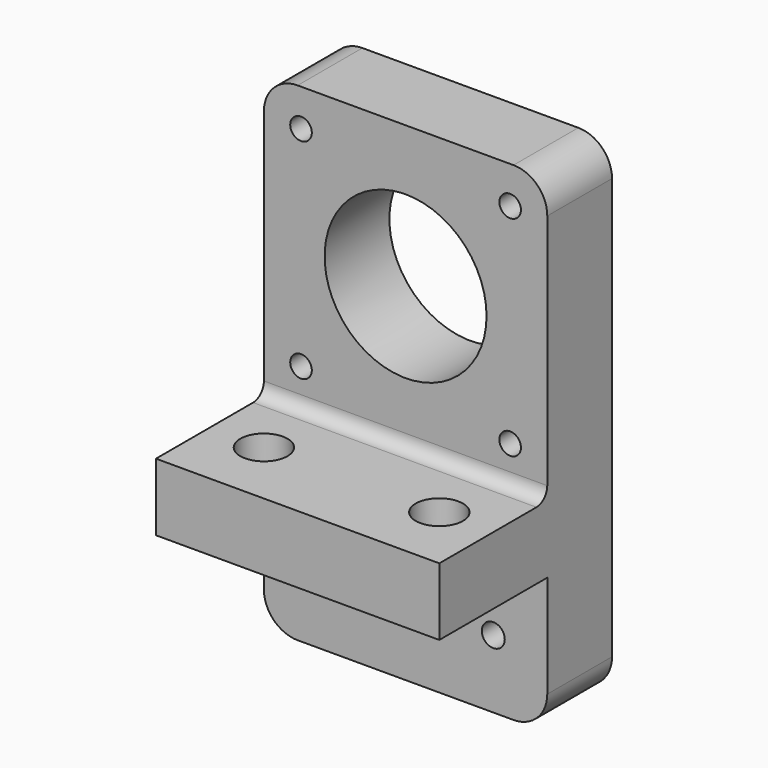
from build123d import *

# Parameters (mm, degrees)
F0_W     = 42
F0_H     = 10
F1_DEPTH = 20
F0_H_2   = 42
F0_R     = 1.6
F0_R_2   = 12
F0_H_3   = 20.2
F0_R_3   = 3.5
F0_H_4   = 0.1999993771
F2_DEPTH = 12
F3_R     = 1.7
F4_DEPTH = 25
F3_R_2   = 3.5
F5_DEPTH = 4
F0_R_4   = 1.7
F6_DEPTH = 12
F7_R     = 3.5
F7_R_2   = 1.7
F8_DEPTH = 2
F9_R     = 5
F10_R    = 2


# Not quite as in the source:
# - a feature names something its author has since deleted; it is built from what else it names


with BuildPart() as f1:
    # F0 (on Front) → F1 (new body)
    with BuildSketch(Plane.XZ):
        with Locations((0, -26.1999993771)):
            Rectangle(F0_W, F0_H)
    extrude(amount=F1_DEPTH)

    # F0 (on Front) → F2 (join)
    with BuildSketch(Plane.XZ):
        Rectangle(F0_W, F0_H_2)
        with Locations((-15.5, -15.5)):
            Circle(F0_R, mode=Mode.SUBTRACT)
        with Locations((15.5, -15.5)):
            Circle(F0_R, mode=Mode.SUBTRACT)
        with Locations((-15.5, 15.5)):
            Circle(F0_R, mode=Mode.SUBTRACT)
        Circle(F0_R_2, mode=Mode.SUBTRACT)
        with Locations((15.5, 15.5)):
            Circle(F0_R, mode=Mode.SUBTRACT)
        with Locations((0, -26.1999993771)):
            Rectangle(F0_W, F0_H)
        with Locations((0, -41.2999993771)):
            Rectangle(F0_W, F0_H_3)
        with Locations((-13, -41.2999993771)):
            Circle(F0_R_3, mode=Mode.SUBTRACT)
        with Locations((13, -41.2999993771)):
            Circle(F0_R_3, mode=Mode.SUBTRACT)
        with Locations((0, -21.0999996886)):
            Rectangle(F0_W, F0_H_4)
    extrude(amount=-F2_DEPTH)

    # F3 (on face) → F4 (cut)
    with BuildSketch(Plane.XY.offset(-21.1999993771)):
        with Locations((-13, -10)):
            Circle(F3_R)
        with Locations((13, -10)):
            Circle(F3_R)
    extrude(amount=-F4_DEPTH, mode=Mode.SUBTRACT)

    # F3 (on face) → F5 (cut)
    with BuildSketch(Plane.XY.offset(-21.1999993771)):
        with Locations((-13, -10)):
            Circle(F3_R_2)
        with Locations((-13, -10)):
            Circle(F3_R, mode=Mode.SUBTRACT)
        with Locations((13, -10)):
            Circle(F3_R_2)
        with Locations((13, -10)):
            Circle(F3_R, mode=Mode.SUBTRACT)
    extrude(amount=-F5_DEPTH, mode=Mode.SUBTRACT)

    # F0 (on Front) → F6 (join)
    with BuildSketch(Plane.XZ):
        with Locations((13, -41.2999993771)):
            Circle(F0_R_3)
        with Locations((13, -41.2999993771)):
            Circle(F0_R_4, mode=Mode.SUBTRACT)
        with Locations((-13, -41.2999993771)):
            Circle(F0_R_3)
        with Locations((-13, -41.2999993771)):
            Circle(F0_R_4, mode=Mode.SUBTRACT)
    extrude(amount=-F6_DEPTH)

    # F7 (on face) → F8 (cut)
    with BuildSketch(Plane(origin=(0, 12, 0), x_dir=(-1, 0, 0), z_dir=(0, 1, 0))):
        with Locations((-13, -41.2999993771)):
            Circle(F7_R)
        with Locations((-13, -41.2999993771)):
            Circle(F7_R_2, mode=Mode.SUBTRACT)
        with Locations((13, -41.2999993771)):
            Circle(F7_R)
        with Locations((13, -41.2999993771)):
            Circle(F7_R_2, mode=Mode.SUBTRACT)
    extrude(amount=-F8_DEPTH, mode=Mode.SUBTRACT)

    # F9
    f9_edges = [f1.edges().sort_by_distance(p)[0] for p in [
        (21, 6, 21),
        (-21, 6, 21),
        (-21, 6, -51.399999),
        (21, 6, -51.399999),
    ]]
    fillet(f9_edges, radius=F9_R)

    # F10
    f10_edges = [f1.edges().sort_by_distance(p)[0] for p in [
        (0, 0, -21.199999),
    ]]
    fillet(f10_edges, radius=F10_R)


solid = f1.part
